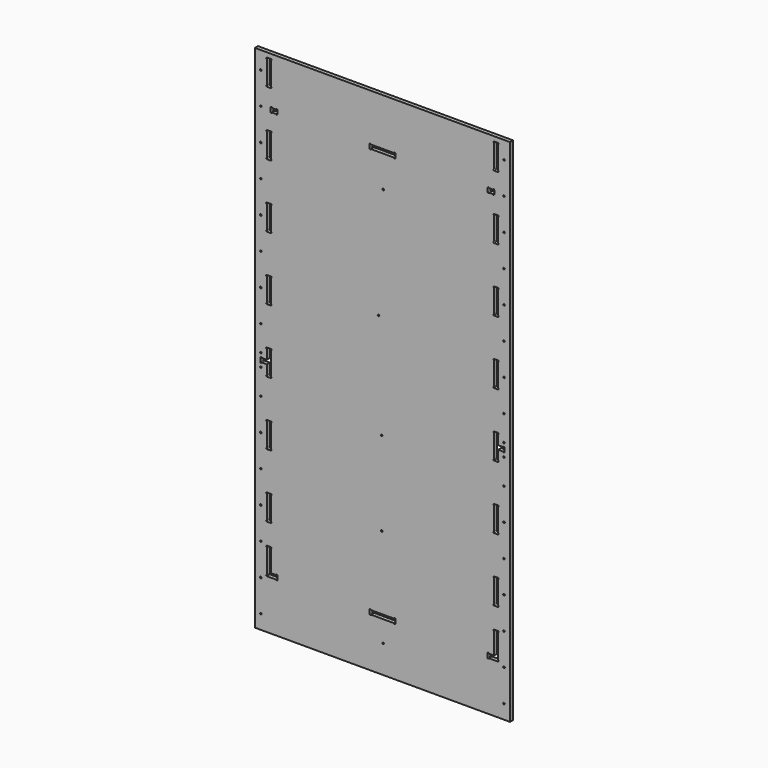
from build123d import *

# Parameters (mm, degrees)
F1_DEPTH = 18


# Not quite as in the source:
# - ends of sketch curves that miss each other by under 0.0002 mm in the source are joined


with BuildPart() as f1:
    # F0 (on Front) → F1 (new body)
    with BuildSketch(Plane.XZ):
        Polygon((-600, 1199.516802), (-600, -1200), (599.475083, -1200), (599.501014, 1199.503749), align=None)
        with BuildLine():
            ThreePointArc((-572.054616, -1136.852261), (-574.7062664294, -1135.7539114294), (-575.804616, -1133.102261))
            ThreePointArc((-575.804616, -1133.102261), (-574.7062664294, -1130.4506105706), (-572.054616, -1129.352261))
            ThreePointArc((-572.054616, -1129.352261), (-569.4029655706, -1130.4506105706), (-568.304616, -1133.102261))
            ThreePointArc((-568.304616, -1133.102261), (-569.4029655706, -1135.7539114294), (-572.054616, -1136.852261))
        make_face(mode=Mode.SUBTRACT)
        with BuildLine():
            ThreePointArc((-572.054616, -986.852261), (-574.7062664294, -985.7539114294), (-575.804616, -983.102261))
            ThreePointArc((-575.804616, -983.102261), (-574.7062664294, -980.4506105706), (-572.054616, -979.352261))
            ThreePointArc((-572.054616, -979.352261), (-569.4029655706, -980.4506105706), (-568.304616, -983.102261))
            ThreePointArc((-568.304616, -983.102261), (-569.4029655706, -985.7539114294), (-572.054616, -986.852261))
        make_face(mode=Mode.SUBTRACT)
        with BuildLine():
            ThreePointArc((-543.7722930308, -848.4810704015), (-546.7808601253, -845.1050301398), (-543.522222, -841.9696830491))
            Line((-543.522222, -841.9696830491), (-525.022204, -841.969884))
            ThreePointArc((-525.022204, -841.969884), (-521.7646201932, -845.1053392321), (-524.7722740702, -848.4812760883))
            Line((-524.7722740702, -848.4812760883), (-524.773356, -949.737518))
            Line((-524.773356, -949.737518), (-500.284715, -949.737785))
            ThreePointArc((-500.284715, -949.737785), (-496.9086751398, -946.7292178747), (-493.7733280491, -949.987856))
            Line((-493.7733280491, -949.987856), (-493.773529, -968.487871))
            ThreePointArc((-493.773529, -968.487871), (-496.9089846919, -971.7454548244), (-500.284921159, -968.7378000122))
            Line((-500.284921159, -968.7378000122), (-543.523601, -968.73733))
            ThreePointArc((-543.523601, -968.73733), (-546.7811848068, -965.6018747679), (-543.7735309298, -962.2259379117))
            Line((-543.7735309298, -962.2259379117), (-543.7722930308, -848.4810704015))
        make_face(mode=Mode.SUBTRACT)
        with BuildLine():
            ThreePointArc((-572.054616, -836.852261), (-574.7062664294, -835.7539114294), (-575.804616, -833.102261))
            ThreePointArc((-575.804616, -833.102261), (-574.7062664294, -830.4506105706), (-572.054616, -829.352261))
            ThreePointArc((-572.054616, -829.352261), (-569.4029655706, -830.4506105706), (-568.304616, -833.102261))
            ThreePointArc((-568.304616, -833.102261), (-569.4029655706, -835.7539114294), (-572.054616, -836.852261))
        make_face(mode=Mode.SUBTRACT)
        with BuildLine():
            ThreePointArc((-572.054616, -686.852261), (-574.7062664294, -685.7539114294), (-575.804616, -683.102261))
            ThreePointArc((-575.804616, -683.102261), (-574.7062664294, -680.4506105706), (-572.054616, -679.352261))
            ThreePointArc((-572.054616, -679.352261), (-569.4029655706, -680.4506105706), (-568.304616, -683.102261))
            ThreePointArc((-568.304616, -683.102261), (-569.4029655706, -685.7539114294), (-572.054616, -686.852261))
        make_face(mode=Mode.SUBTRACT)
        with BuildLine():
            ThreePointArc((-525.019977, -621.9649860431), (-521.7623931741, -625.1004417303), (-524.7700480643, -628.4763781649))
            Line((-524.7700480643, -628.4763781649), (-524.771223, -736.453766))
            ThreePointArc((-524.771223, -736.453766), (-521.7626558747, -739.8298058602), (-525.021294, -742.9651529509))
            Line((-525.021294, -742.9651529509), (-543.521145, -742.964956))
            ThreePointArc((-543.521145, -742.964956), (-546.7787288244, -739.8295003081), (-543.7710740122, -736.453563841))
            Line((-543.7710740122, -736.453563841), (-543.769899, -628.476172))
            ThreePointArc((-543.769899, -628.476172), (-546.7784661253, -625.1001321398), (-543.519828, -621.9647850491))
            Line((-543.519828, -621.9647850491), (-525.019977, -621.9649860431))
        make_face(mode=Mode.SUBTRACT)
        with BuildLine():
            ThreePointArc((-60.7727499569, -949.992565), (-57.6372943081, -946.7349811756), (-54.261357841, -949.7426359878))
            Line((-54.261357841, -949.7426359878), (53.715983, -949.743811))
            ThreePointArc((53.715983, -949.743811), (57.0920228602, -946.7352438747), (60.2273699509, -949.993882))
            Line((60.2273699509, -949.993882), (60.227168, -968.4939))
            ThreePointArc((60.227168, -968.4939), (57.0917123081, -971.7514838244), (53.715775841, -968.7438290122))
            Line((53.715775841, -968.7438290122), (-54.261565, -968.742654))
            ThreePointArc((-54.261565, -968.742654), (-57.6376048602, -971.7512211253), (-60.7729519509, -968.492583))
            Line((-60.7729519509, -968.492583), (-60.7727499569, -949.992565))
        make_face(mode=Mode.SUBTRACT)
        with BuildLine():
            ThreePointArc((-8.115127, -606.325), (-7.0167774294, -603.6733495706), (-4.365127, -602.575))
            ThreePointArc((-4.365127, -602.575), (-1.7134765706, -603.6733495706), (-0.615127, -606.325))
            ThreePointArc((-0.615127, -606.325), (-1.7134765706, -608.9766504294), (-4.365127, -610.075))
            ThreePointArc((-4.365127, -610.075), (-7.0167774294, -608.9766504294), (-8.115127, -606.325))
        make_face(mode=Mode.SUBTRACT)
        with BuildLine():
            ThreePointArc((-572.054616, -536.852261), (-574.7062664294, -535.7539114294), (-575.804616, -533.102261))
            ThreePointArc((-575.804616, -533.102261), (-574.7062664294, -530.4506105706), (-572.054616, -529.352261))
            ThreePointArc((-572.054616, -529.352261), (-569.4029655706, -530.4506105706), (-568.304616, -533.102261))
            ThreePointArc((-568.304616, -533.102261), (-569.4029655706, -535.7539114294), (-572.054616, -536.852261))
        make_face(mode=Mode.SUBTRACT)
        with BuildLine():
            ThreePointArc((-572.054616, -386.852261), (-574.7062664294, -385.7539114294), (-575.804616, -383.102261))
            ThreePointArc((-575.804616, -383.102261), (-574.7062664294, -380.4506105706), (-572.054616, -379.352261))
            ThreePointArc((-572.054616, -379.352261), (-569.4029655706, -380.4506105706), (-568.304616, -383.102261))
            ThreePointArc((-568.304616, -383.102261), (-569.4029655706, -385.7539114294), (-572.054616, -386.852261))
        make_face(mode=Mode.SUBTRACT)
        with BuildLine():
            ThreePointArc((-525.016712, -321.9646860431), (-521.7591281741, -325.1001417303), (-524.7667830643, -328.4760781649))
            Line((-524.7667830643, -328.4760781649), (-524.767958, -436.453466))
            ThreePointArc((-524.767958, -436.453466), (-521.7593908747, -439.8295058602), (-525.018029, -442.9648529509))
            Line((-525.018029, -442.9648529509), (-543.51788, -442.964656))
            ThreePointArc((-543.51788, -442.964656), (-546.7754638244, -439.8292003081), (-543.7678090122, -436.453263841))
            Line((-543.7678090122, -436.453263841), (-543.766634, -328.475872))
            ThreePointArc((-543.766634, -328.475872), (-546.7752011253, -325.0998321398), (-543.516563, -321.9644850491))
            Line((-543.516563, -321.9644850491), (-525.016712, -321.9646860431))
        make_face(mode=Mode.SUBTRACT)
        with BuildLine():
            ThreePointArc((-572.054616, -236.852261), (-574.7062664294, -235.7539114294), (-575.804616, -233.102261))
            ThreePointArc((-575.804616, -233.102261), (-574.7062664294, -230.4506105706), (-572.054616, -229.352261))
            ThreePointArc((-572.054616, -229.352261), (-569.4029655706, -230.4506105706), (-568.304616, -233.102261))
            ThreePointArc((-568.304616, -233.102261), (-569.4029655706, -235.7539114294), (-572.054616, -236.852261))
        make_face(mode=Mode.SUBTRACT)
        with BuildLine():
            ThreePointArc((-572.054616, -116.852261), (-574.7062664294, -115.7539114294), (-575.804616, -113.102261))
            ThreePointArc((-575.804616, -113.102261), (-574.7062664294, -110.4506105706), (-572.054616, -109.352261))
            ThreePointArc((-572.054616, -109.352261), (-569.4029655706, -110.4506105706), (-568.304616, -113.102261))
            ThreePointArc((-568.304616, -113.102261), (-569.4029655706, -115.7539114294), (-572.054616, -116.852261))
        make_face(mode=Mode.SUBTRACT)
        with BuildLine():
            ThreePointArc((-543.514634, -142.9690389274), (-546.7720658527, -139.8334261548), (-543.7642489368, -136.4576348202))
            Line((-543.7642489368, -136.4576348202), (-543.76158, -91.971957))
            Line((-543.76158, -91.971957), (-568.250197, -91.971691))
            ThreePointArc((-568.250197, -91.971691), (-571.6262368602, -94.9802581253), (-574.7615839509, -91.72162))
            Line((-574.7615839509, -91.72162), (-574.761383, -73.221602))
            ThreePointArc((-574.761383, -73.221602), (-571.6259272697, -69.9640181741), (-568.2499908351, -72.9716730643))
            Line((-568.2499908351, -72.9716730643), (-543.761373, -72.971939))
            Line((-543.761373, -72.971939), (-543.763074, -28.480267))
            ThreePointArc((-543.763074, -28.480267), (-546.7718041555, -25.1043722531), (-543.513317, -21.9688680257))
            Line((-543.513317, -21.9688680257), (-525.013448, -21.969069))
            ThreePointArc((-525.013448, -21.969069), (-521.7558641756, -25.1045246919), (-524.7635189878, -28.480461159))
            Line((-524.7635189878, -28.480461159), (-524.764694, -136.457849))
            ThreePointArc((-524.764694, -136.457849), (-521.7561268747, -139.8338888602), (-525.014765, -142.9692359509))
            Line((-525.014765, -142.9692359509), (-543.514634, -142.9690389274))
        make_face(mode=Mode.SUBTRACT)
        with BuildLine():
            ThreePointArc((-572.054616, -56.852261), (-574.7062664294, -55.7539114294), (-575.804616, -53.102261))
            ThreePointArc((-575.804616, -53.102261), (-574.7062664294, -50.4506105706), (-572.054616, -49.352261))
            ThreePointArc((-572.054616, -49.352261), (-569.4029655706, -50.4506105706), (-568.304616, -53.102261))
            ThreePointArc((-568.304616, -53.102261), (-569.4029655706, -55.7539114294), (-572.054616, -56.852261))
        make_face(mode=Mode.SUBTRACT)
        with BuildLine():
            ThreePointArc((-8.115127, -210.239), (-7.0167774294, -207.5873495706), (-4.365127, -206.489))
            ThreePointArc((-4.365127, -206.489), (-1.7134765706, -207.5873495706), (-0.615127, -210.239))
            ThreePointArc((-0.615127, -210.239), (-1.7134765706, -212.8906504294), (-4.365127, -213.989))
            ThreePointArc((-4.365127, -213.989), (-7.0167774294, -212.8906504294), (-8.115127, -210.239))
        make_face(mode=Mode.SUBTRACT)
        with BuildLine():
            ThreePointArc((-0.780127, -1068.426), (0.3182225706, -1065.7743495706), (2.969873, -1064.676))
            ThreePointArc((2.969873, -1064.676), (5.6215234294, -1065.7743495706), (6.719873, -1068.426))
            ThreePointArc((6.719873, -1068.426), (5.6215234294, -1071.0776504294), (2.969873, -1072.176))
            ThreePointArc((2.969873, -1072.176), (0.3182225706, -1071.0776504294), (-0.780127, -1068.426))
        make_face(mode=Mode.SUBTRACT)
        with BuildLine():
            ThreePointArc((571.095767, -1136.852261), (568.4441165706, -1135.7539114294), (567.345767, -1133.102261))
            ThreePointArc((567.345767, -1133.102261), (568.4441165706, -1130.4506105706), (571.095767, -1129.352261))
            ThreePointArc((571.095767, -1129.352261), (573.7474174294, -1130.4506105706), (574.845767, -1133.102261))
            ThreePointArc((574.845767, -1133.102261), (573.7474174294, -1135.7539114294), (571.095767, -1136.852261))
        make_face(mode=Mode.SUBTRACT)
        with BuildLine():
            ThreePointArc((524.2286739692, -848.4939214015), (521.2201068747, -845.1178811398), (524.478745, -841.9825340491))
            Line((524.478745, -841.9825340491), (542.979136, -841.982735))
            ThreePointArc((542.979136, -841.982735), (546.2367198259, -845.1181907303), (543.2290649357, -848.4941271649))
            Line((543.2290649357, -848.4941271649), (543.227828, -962.237769))
            ThreePointArc((543.227828, -962.237769), (546.2363951253, -965.6138088602), (542.977757, -968.7491559509))
            Line((542.977757, -968.7491559509), (499.738725, -968.748685))
            ThreePointArc((499.738725, -968.748685), (496.3626841781, -971.7572521267), (493.2273370491, -968.498614))
            Line((493.2273370491, -968.498614), (493.227539, -949.998596))
            ThreePointArc((493.227539, -949.998596), (496.3629946919, -946.7410121756), (499.738931159, -949.7486669878))
            Line((499.738931159, -949.7486669878), (524.227573, -949.748934))
            Line((524.227573, -949.748934), (524.2286739692, -848.4939214015))
        make_face(mode=Mode.SUBTRACT)
        with BuildLine():
            ThreePointArc((571.095767, -986.852261), (568.4441165706, -985.7539114294), (567.345767, -983.102261))
            ThreePointArc((567.345767, -983.102261), (568.4441165706, -980.4506105706), (571.095767, -979.352261))
            ThreePointArc((571.095767, -979.352261), (573.7474174294, -980.4506105706), (574.845767, -983.102261))
            ThreePointArc((574.845767, -983.102261), (573.7474174294, -985.7539114294), (571.095767, -986.852261))
        make_face(mode=Mode.SUBTRACT)
        with BuildLine():
            ThreePointArc((571.095767, -836.852261), (568.4441165706, -835.7539114294), (567.345767, -833.102261))
            ThreePointArc((567.345767, -833.102261), (568.4441165706, -830.4506105706), (571.095767, -829.352261))
            ThreePointArc((571.095767, -829.352261), (573.7474174294, -830.4506105706), (574.845767, -833.102261))
            ThreePointArc((574.845767, -833.102261), (573.7474174294, -835.7539114294), (571.095767, -836.852261))
        make_face(mode=Mode.SUBTRACT)
        with BuildLine():
            Line((524.230052, -736.46863), (524.231227, -628.49129))
            ThreePointArc((524.231227, -628.49129), (521.2226598747, -625.1152501398), (524.481298, -621.9799030491))
            Line((524.481298, -621.9799030491), (542.981316, -621.980104))
            ThreePointArc((542.981316, -621.980104), (546.2388998259, -625.1155597303), (543.2312449357, -628.4914961649))
            Line((543.2312449357, -628.4914961649), (543.23007, -736.468837))
            ThreePointArc((543.23007, -736.468837), (546.2386371253, -739.8448768602), (542.979999, -742.9802239509))
            Line((542.979999, -742.9802239509), (524.479981, -742.980023))
            ThreePointArc((524.479981, -742.980023), (521.2223971741, -739.8445672697), (524.230052, -736.46863))
        make_face(mode=Mode.SUBTRACT)
        with BuildLine():
            ThreePointArc((571.095767, -686.852261), (568.4441165706, -685.7539114294), (567.345767, -683.102261))
            ThreePointArc((567.345767, -683.102261), (568.4441165706, -680.4506105706), (571.095767, -679.352261))
            ThreePointArc((571.095767, -679.352261), (573.7474174294, -680.4506105706), (574.845767, -683.102261))
            ThreePointArc((574.845767, -683.102261), (573.7474174294, -685.7539114294), (571.095767, -686.852261))
        make_face(mode=Mode.SUBTRACT)
        with BuildLine():
            ThreePointArc((571.095767, -536.852261), (568.4441165706, -535.7539114294), (567.345767, -533.102261))
            ThreePointArc((567.345767, -533.102261), (568.4441165706, -530.4506105706), (571.095767, -529.352261))
            ThreePointArc((571.095767, -529.352261), (573.7474174294, -530.4506105706), (574.845767, -533.102261))
            ThreePointArc((574.845767, -533.102261), (573.7474174294, -535.7539114294), (571.095767, -536.852261))
        make_face(mode=Mode.SUBTRACT)
        with BuildLine():
            ThreePointArc((524.483246, -442.9797229569), (521.2256621741, -439.8442672697), (524.2333170643, -436.4683308351))
            Line((524.2333170643, -436.4683308351), (524.234492, -328.49099))
            ThreePointArc((524.234492, -328.49099), (521.2259238556, -325.114950638), (524.484562, -321.9796030491))
            Line((524.484562, -321.9796030491), (542.98458, -321.979804))
            ThreePointArc((542.98458, -321.979804), (546.2421638068, -325.1152592321), (543.2345099298, -328.4911960883))
            Line((543.2345099298, -328.4911960883), (543.233335, -436.468537))
            ThreePointArc((543.233335, -436.468537), (546.2419021253, -439.8445768602), (542.983264, -442.9799239509))
            Line((542.983264, -442.9799239509), (524.483246, -442.9797229569))
        make_face(mode=Mode.SUBTRACT)
        with BuildLine():
            ThreePointArc((571.095767, -386.852261), (568.4441165706, -385.7539114294), (567.345767, -383.102261))
            ThreePointArc((567.345767, -383.102261), (568.4441165706, -380.4506105706), (571.095767, -379.352261))
            ThreePointArc((571.095767, -379.352261), (573.7474174294, -380.4506105706), (574.845767, -383.102261))
            ThreePointArc((574.845767, -383.102261), (573.7474174294, -385.7539114294), (571.095767, -386.852261))
        make_face(mode=Mode.SUBTRACT)
        with BuildLine():
            ThreePointArc((571.095767, -236.852261), (568.4441165706, -235.7539114294), (567.345767, -233.102261))
            ThreePointArc((567.345767, -233.102261), (568.4441165706, -230.4506105706), (571.095767, -229.352261))
            ThreePointArc((571.095767, -229.352261), (573.7474174294, -230.4506105706), (574.845767, -233.102261))
            ThreePointArc((574.845767, -233.102261), (573.7474174294, -235.7539114294), (571.095767, -236.852261))
        make_face(mode=Mode.SUBTRACT)
        with BuildLine():
            ThreePointArc((524.2377559692, -28.4906904015), (521.2291888747, -25.1146501398), (524.487827, -21.9793030491))
            Line((524.487827, -21.9793030491), (542.987819, -21.979504))
            ThreePointArc((542.987819, -21.979504), (546.2456103474, -25.1147390342), (543.238188986, -28.4908788184))
            Line((543.238188986, -28.4908788184), (543.240772, -72.983768))
            Line((543.240772, -72.983768), (567.729447, -72.984035))
            ThreePointArc((567.729447, -72.984035), (571.105486362, -69.9754668556), (574.2408339509, -73.234105))
            Line((574.2408339509, -73.234105), (574.240633, -91.734123))
            ThreePointArc((574.240633, -91.734123), (571.1051778062, -94.9917068053), (567.7292409176, -91.9840530063))
            Line((567.7292409176, -91.9840530063), (543.240565, -91.983786))
            Line((543.240565, -91.983786), (543.237014, -136.468254))
            ThreePointArc((543.237014, -136.468254), (546.2453486433, -139.8444975193), (542.986502, -142.979623906))
            Line((542.986502, -142.979623906), (524.48651, -142.979423))
            ThreePointArc((524.48651, -142.979423), (521.2289261741, -139.8439672697), (524.2365810643, -136.4680308351))
            Line((524.2365810643, -136.4680308351), (524.2377559692, -28.4906904015))
        make_face(mode=Mode.SUBTRACT)
        with BuildLine():
            ThreePointArc((571.095767, -116.852261), (568.4441165706, -115.7539114294), (567.345767, -113.102261))
            ThreePointArc((567.345767, -113.102261), (568.4441165706, -110.4506105706), (571.095767, -109.352261))
            ThreePointArc((571.095767, -109.352261), (573.7474174294, -110.4506105706), (574.845767, -113.102261))
            ThreePointArc((574.845767, -113.102261), (573.7474174294, -115.7539114294), (571.095767, -116.852261))
        make_face(mode=Mode.SUBTRACT)
        with BuildLine():
            ThreePointArc((571.095767, -56.852261), (568.4441165706, -55.7539114294), (567.345767, -53.102261))
            ThreePointArc((567.345767, -53.102261), (568.4441165706, -50.4506105706), (571.095767, -49.352261))
            ThreePointArc((571.095767, -49.352261), (573.7474174294, -50.4506105706), (574.845767, -53.102261))
            ThreePointArc((574.845767, -53.102261), (573.7474174294, -55.7539114294), (571.095767, -56.852261))
        make_face(mode=Mode.SUBTRACT)
        with BuildLine():
            ThreePointArc((-572.054616, 63.147739), (-574.7062664294, 64.2460885706), (-575.804616, 66.897739))
            ThreePointArc((-575.804616, 66.897739), (-574.7062664294, 69.5493894294), (-572.054616, 70.647739))
            ThreePointArc((-572.054616, 70.647739), (-569.4029655706, 69.5493894294), (-568.304616, 66.897739))
            ThreePointArc((-568.304616, 66.897739), (-569.4029655706, 64.2460885706), (-572.054616, 63.147739))
        make_face(mode=Mode.SUBTRACT)
        with BuildLine():
            ThreePointArc((-572.054616, 213.147739), (-574.7062664294, 214.2460885706), (-575.804616, 216.897739))
            ThreePointArc((-575.804616, 216.897739), (-574.7062664294, 219.5493894294), (-572.054616, 220.647739))
            ThreePointArc((-572.054616, 220.647739), (-569.4029655706, 219.5493894294), (-568.304616, 216.897739))
            ThreePointArc((-568.304616, 216.897739), (-569.4029655706, 214.2460885706), (-572.054616, 213.147739))
        make_face(mode=Mode.SUBTRACT)
        with BuildLine():
            ThreePointArc((-524.7614289692, 163.5471344015), (-521.7528618747, 160.1710941398), (-525.0115, 157.0357470491))
            Line((-525.0115, 157.0357470491), (-543.511351, 157.035943))
            ThreePointArc((-543.511351, 157.035943), (-546.7689348259, 160.1713987303), (-543.7612799357, 163.5473351649))
            Line((-543.7612799357, 163.5473351649), (-543.760105, 271.524728))
            ThreePointArc((-543.760105, 271.524728), (-546.7686721253, 274.9007678602), (-543.510034, 278.0361149509))
            Line((-543.510034, 278.0361149509), (-525.010183, 278.035914))
            ThreePointArc((-525.010183, 278.035914), (-521.7525991741, 274.9004582697), (-524.7602540643, 271.5245218351))
            Line((-524.7602540643, 271.5245218351), (-524.7614289692, 163.5471344015))
        make_face(mode=Mode.SUBTRACT)
        with BuildLine():
            ThreePointArc((-572.054616, 363.147739), (-574.7062664294, 364.2460885706), (-575.804616, 366.897739))
            ThreePointArc((-575.804616, 366.897739), (-574.7062664294, 369.5493894294), (-572.054616, 370.647739))
            ThreePointArc((-572.054616, 370.647739), (-569.4029655706, 369.5493894294), (-568.304616, 366.897739))
            ThreePointArc((-568.304616, 366.897739), (-569.4029655706, 364.2460885706), (-572.054616, 363.147739))
        make_face(mode=Mode.SUBTRACT)
        with BuildLine():
            ThreePointArc((-572.054616, 513.147739), (-574.7062664294, 514.2460885706), (-575.804616, 516.897739))
            ThreePointArc((-575.804616, 516.897739), (-574.7062664294, 519.5493894294), (-572.054616, 520.647739))
            ThreePointArc((-572.054616, 520.647739), (-569.4029655706, 519.5493894294), (-568.304616, 516.897739))
            ThreePointArc((-568.304616, 516.897739), (-569.4029655706, 514.2460885706), (-572.054616, 513.147739))
        make_face(mode=Mode.SUBTRACT)
        with BuildLine():
            ThreePointArc((-525.006919, 578.0362139569), (-521.7493351932, 574.9007587679), (-524.7569890702, 571.5248219117))
            Line((-524.7569890702, 571.5248219117), (-524.758164, 463.547434))
            ThreePointArc((-524.758164, 463.547434), (-521.7495968747, 460.1713941398), (-525.008235, 457.0360470491))
            Line((-525.008235, 457.0360470491), (-543.508086, 457.036243))
            ThreePointArc((-543.508086, 457.036243), (-546.7656698259, 460.1716987303), (-543.7580149357, 463.5476351649))
            Line((-543.7580149357, 463.5476351649), (-543.75684, 571.525028))
            ThreePointArc((-543.75684, 571.525028), (-546.7654081444, 574.901067362), (-543.50677, 578.0364149509))
            Line((-543.50677, 578.0364149509), (-525.006919, 578.0362139569))
        make_face(mode=Mode.SUBTRACT)
        with BuildLine():
            ThreePointArc((-22.784127, 281.201), (-21.6857774294, 283.8526504294), (-19.034127, 284.951))
            ThreePointArc((-19.034127, 284.951), (-16.3824765706, 283.8526504294), (-15.284127, 281.201))
            ThreePointArc((-15.284127, 281.201), (-16.3824765706, 278.5493495706), (-19.034127, 277.451))
            ThreePointArc((-19.034127, 277.451), (-21.6857774294, 278.5493495706), (-22.784127, 281.201))
        make_face(mode=Mode.SUBTRACT)
        with BuildLine():
            ThreePointArc((-572.054616, 663.147739), (-574.7062664294, 664.2460885706), (-575.804616, 666.897739))
            ThreePointArc((-575.804616, 666.897739), (-574.7062664294, 669.5493894294), (-572.054616, 670.647739))
            ThreePointArc((-572.054616, 670.647739), (-569.4029655706, 669.5493894294), (-568.304616, 666.897739))
            ThreePointArc((-568.304616, 666.897739), (-569.4029655706, 664.2460885706), (-572.054616, 663.147739))
        make_face(mode=Mode.SUBTRACT)
        with BuildLine():
            ThreePointArc((-572.054616, 813.147739), (-574.7062664294, 814.2460885706), (-575.804616, 816.897739))
            ThreePointArc((-575.804616, 816.897739), (-574.7062664294, 819.5493894294), (-572.054616, 820.647739))
            ThreePointArc((-572.054616, 820.647739), (-569.4029655706, 819.5493894294), (-568.304616, 816.897739))
            ThreePointArc((-568.304616, 816.897739), (-569.4029655706, 814.2460885706), (-572.054616, 813.147739))
        make_face(mode=Mode.SUBTRACT)
        with BuildLine():
            ThreePointArc((-543.7533610308, 871.5253315985), (-546.7619281253, 874.9013718602), (-543.50329, 878.0367189509))
            Line((-543.50329, 878.0367189509), (-525.003272, 878.036518))
            ThreePointArc((-525.003272, 878.036518), (-521.7456881741, 874.9010622697), (-524.7533430643, 871.5251258351))
            Line((-524.7533430643, 871.5251258351), (-524.754518, 763.547734))
            ThreePointArc((-524.754518, 763.547734), (-521.7459508747, 760.1716941398), (-525.004589, 757.0363470491))
            Line((-525.004589, 757.0363470491), (-543.504607, 757.036548))
            ThreePointArc((-543.504607, 757.036548), (-546.7621908244, 760.1720036919), (-543.7545360122, 763.547940159))
            Line((-543.7545360122, 763.547940159), (-543.7533610308, 871.5253315985))
        make_face(mode=Mode.SUBTRACT)
        with BuildLine():
            ThreePointArc((-572.054616, 963.147739), (-574.7062664294, 964.2460885706), (-575.804616, 966.897739))
            ThreePointArc((-575.804616, 966.897739), (-574.7062664294, 969.5493894294), (-572.054616, 970.647739))
            ThreePointArc((-572.054616, 970.647739), (-569.4029655706, 969.5493894294), (-568.304616, 966.897739))
            ThreePointArc((-568.304616, 966.897739), (-569.4029655706, 964.2460885706), (-572.054616, 963.147739))
        make_face(mode=Mode.SUBTRACT)
        with BuildLine():
            ThreePointArc((-501.2644784015, 977.0329490308), (-497.8884391391, 980.0415161637), (-494.7530910488, 976.78288))
            Line((-494.7530910488, 976.78288), (-494.752949, 958.277954))
            ThreePointArc((-494.752949, 958.277954), (-497.888403196, 955.0203682323), (-501.2643420088, 958.0280219993))
            Line((-501.2643420088, 958.0280219993), (-519.241595, 958.028218))
            ThreePointArc((-519.241595, 958.028218), (-522.6176343606, 955.0196508555), (-525.752981951, 958.278288))
            Line((-525.752981951, 958.278288), (-525.752923, 976.783214))
            ThreePointArc((-525.752923, 976.783214), (-522.6174677679, 980.0407978068), (-519.2415309117, 977.0331439298))
            Line((-519.2415309117, 977.0331439298), (-501.2644784015, 977.0329490308))
        make_face(mode=Mode.SUBTRACT)
        with BuildLine():
            ThreePointArc((-572.054616, 1113.147739), (-574.7062664294, 1114.2460885706), (-575.804616, 1116.897739))
            ThreePointArc((-575.804616, 1116.897739), (-574.7062664294, 1119.5493894294), (-572.054616, 1120.647739))
            ThreePointArc((-572.054616, 1120.647739), (-569.4029655706, 1119.5493894294), (-568.304616, 1116.897739))
            ThreePointArc((-568.304616, 1116.897739), (-569.4029655706, 1114.2460885706), (-572.054616, 1113.147739))
        make_face(mode=Mode.SUBTRACT)
        with BuildLine():
            ThreePointArc((-524.7515879633, 1063.5478364778), (-521.7430198556, 1060.171796638), (-525.001658, 1057.0364490491))
            Line((-525.001658, 1057.0364490491), (-543.501509, 1057.036651))
            ThreePointArc((-543.501509, 1057.036651), (-546.7590928244, 1060.1721066919), (-543.7514380122, 1063.548043159))
            Line((-543.7514380122, 1063.548043159), (-543.750263, 1171.525431))
            ThreePointArc((-543.750263, 1171.525431), (-546.7588311444, 1174.901470362), (-543.500193, 1178.0368179509))
            Line((-543.500193, 1178.0368179509), (-525.000342, 1178.036621))
            ThreePointArc((-525.000342, 1178.036621), (-521.7427581932, 1174.9011657679), (-524.7504120702, 1171.5252289117))
            Line((-524.7504120702, 1171.5252289117), (-524.7515879633, 1063.5478364778))
        make_face(mode=Mode.SUBTRACT)
        with BuildLine():
            ThreePointArc((53.7365535985, 977.0268890308), (57.1125928609, 980.0354561637), (60.2479409512, 976.77682))
            Line((60.2479409512, 976.77682), (60.248139, 958.276642))
            ThreePointArc((60.248139, 958.276642), (57.1126843059, 955.0190572139), (53.7367469176, 958.0267109937))
            Line((53.7367469176, 958.0267109937), (-54.240597, 958.027886))
            ThreePointArc((-54.240597, 958.027886), (-57.6166358624, 955.0193178364), (-60.751983951, 958.277955))
            Line((-60.751983951, 958.277955), (-60.751982, 976.778133))
            ThreePointArc((-60.751982, 976.778133), (-57.6165273059, 980.0357177861), (-54.2405899176, 977.0280640063))
            Line((-54.2405899176, 977.0280640063), (53.7365535985, 977.0268890308))
        make_face(mode=Mode.SUBTRACT)
        with BuildLine():
            ThreePointArc((571.095767, 63.147739), (568.4441165706, 64.2460885706), (567.345767, 66.897739))
            ThreePointArc((567.345767, 66.897739), (568.4441165706, 69.5493894294), (571.095767, 70.647739))
            ThreePointArc((571.095767, 70.647739), (573.7474174294, 69.5493894294), (574.845767, 66.897739))
            ThreePointArc((574.845767, 66.897739), (573.7474174294, 64.2460885706), (571.095767, 63.147739))
        make_face(mode=Mode.SUBTRACT)
        with BuildLine():
            ThreePointArc((524.489775, 157.0208770431), (521.2321911741, 160.1563327303), (524.2398460643, 163.5322691649))
            Line((524.2398460643, 163.5322691649), (524.241021, 271.50961))
            ThreePointArc((524.241021, 271.50961), (521.2324538747, 274.8856498602), (524.491092, 278.0209969509))
            Line((524.491092, 278.0209969509), (542.99111, 278.020796))
            ThreePointArc((542.99111, 278.020796), (546.2486938259, 274.8853402697), (543.2410389357, 271.5094038351))
            Line((543.2410389357, 271.5094038351), (543.239864, 163.532063))
            ThreePointArc((543.239864, 163.532063), (546.2484311253, 160.1560231398), (542.989793, 157.0206760491))
            Line((542.989793, 157.0206760491), (524.489775, 157.0208770431))
        make_face(mode=Mode.SUBTRACT)
        with BuildLine():
            ThreePointArc((571.095767, 213.147739), (568.4441165706, 214.2460885706), (567.345767, 216.897739))
            ThreePointArc((567.345767, 216.897739), (568.4441165706, 219.5493894294), (571.095767, 220.647739))
            ThreePointArc((571.095767, 220.647739), (573.7474174294, 219.5493894294), (574.845767, 216.897739))
            ThreePointArc((574.845767, 216.897739), (573.7474174294, 214.2460885706), (571.095767, 213.147739))
        make_face(mode=Mode.SUBTRACT)
        with BuildLine():
            ThreePointArc((571.095767, 363.147739), (568.4441165706, 364.2460885706), (567.345767, 366.897739))
            ThreePointArc((567.345767, 366.897739), (568.4441165706, 369.5493894294), (571.095767, 370.647739))
            ThreePointArc((571.095767, 370.647739), (573.7474174294, 369.5493894294), (574.845767, 366.897739))
            ThreePointArc((574.845767, 366.897739), (573.7474174294, 364.2460885706), (571.095767, 363.147739))
        make_face(mode=Mode.SUBTRACT)
        with BuildLine():
            ThreePointArc((524.493039, 457.0211770431), (521.2354551741, 460.1566327303), (524.2431100643, 463.5325691649))
            Line((524.2431100643, 463.5325691649), (524.244285, 571.50991))
            ThreePointArc((524.244285, 571.50991), (521.2357178747, 574.8859498602), (524.494356, 578.0212969509))
            Line((524.494356, 578.0212969509), (542.994374, 578.021096))
            ThreePointArc((542.994374, 578.021096), (546.2519578259, 574.8856402697), (543.2443029357, 571.5097038351))
            Line((543.2443029357, 571.5097038351), (543.243128, 463.532363))
            ThreePointArc((543.243128, 463.532363), (546.2516951253, 460.1563231398), (542.993057, 457.0209760491))
            Line((542.993057, 457.0209760491), (524.493039, 457.0211770431))
        make_face(mode=Mode.SUBTRACT)
        with BuildLine():
            ThreePointArc((571.095767, 513.147739), (568.4441165706, 514.2460885706), (567.345767, 516.897739))
            ThreePointArc((567.345767, 516.897739), (568.4441165706, 519.5493894294), (571.095767, 520.647739))
            ThreePointArc((571.095767, 520.647739), (573.7474174294, 519.5493894294), (574.845767, 516.897739))
            ThreePointArc((574.845767, 516.897739), (573.7474174294, 514.2460885706), (571.095767, 513.147739))
        make_face(mode=Mode.SUBTRACT)
        with BuildLine():
            ThreePointArc((-0.780127, 809.315), (0.3182225706, 811.9666504294), (2.969873, 813.065))
            ThreePointArc((2.969873, 813.065), (5.6215234294, 811.9666504294), (6.719873, 809.315))
            ThreePointArc((6.719873, 809.315), (5.6215234294, 806.6633495706), (2.969873, 805.565))
            ThreePointArc((2.969873, 805.565), (0.3182225706, 806.6633495706), (-0.780127, 809.315))
        make_face(mode=Mode.SUBTRACT)
        with BuildLine():
            ThreePointArc((571.095767, 663.147739), (568.4441165706, 664.2460885706), (567.345767, 666.897739))
            ThreePointArc((567.345767, 666.897739), (568.4441165706, 669.5493894294), (571.095767, 670.647739))
            ThreePointArc((571.095767, 670.647739), (573.7474174294, 669.5493894294), (574.845767, 666.897739))
            ThreePointArc((574.845767, 666.897739), (573.7474174294, 664.2460885706), (571.095767, 663.147739))
        make_face(mode=Mode.SUBTRACT)
        with BuildLine():
            ThreePointArc((524.496304, 757.0214770431), (521.2387201741, 760.1569327303), (524.2463750643, 763.5328691649))
            Line((524.2463750643, 763.5328691649), (524.24755, 871.51021))
            ThreePointArc((524.24755, 871.51021), (521.2389828747, 874.8862498602), (524.497621, 878.0215969509))
            Line((524.497621, 878.0215969509), (542.997639, 878.021396))
            ThreePointArc((542.997639, 878.021396), (546.2552228259, 874.8859402697), (543.2475679357, 871.5100038351))
            Line((543.2475679357, 871.5100038351), (543.246393, 763.532663))
            ThreePointArc((543.246393, 763.532663), (546.2549601253, 760.1566231398), (542.996322, 757.0212760491))
            Line((542.996322, 757.0212760491), (524.496304, 757.0214770431))
        make_face(mode=Mode.SUBTRACT)
        with BuildLine():
            ThreePointArc((571.095767, 813.147739), (568.4441165706, 814.2460885706), (567.345767, 816.897739))
            ThreePointArc((567.345767, 816.897739), (568.4441165706, 819.5493894294), (571.095767, 820.647739))
            ThreePointArc((571.095767, 820.647739), (573.7474174294, 819.5493894294), (574.845767, 816.897739))
            ThreePointArc((574.845767, 816.897739), (573.7474174294, 814.2460885706), (571.095767, 813.147739))
        make_face(mode=Mode.SUBTRACT)
        with BuildLine():
            ThreePointArc((525.2483379569, 958.271581), (522.1128827679, 955.0139971932), (518.7369459117, 958.0216510702))
            Line((518.7369459117, 958.0216510702), (500.759692, 958.021846))
            ThreePointArc((500.759692, 958.021846), (497.3836521398, 955.0132788747), (494.2483050491, 958.271917))
            Line((494.2483050491, 958.271917), (494.248523, 976.772078))
            ThreePointArc((494.248523, 976.772078), (497.3839786919, 980.0296618244), (500.759915159, 977.0220070122))
            Line((500.759915159, 977.0220070122), (518.736978, 977.021812))
            ThreePointArc((518.736978, 977.021812), (522.1130173606, 980.0303791445), (525.248364951, 976.771742))
            Line((525.248364951, 976.771742), (525.2483379569, 958.271581))
        make_face(mode=Mode.SUBTRACT)
        with BuildLine():
            ThreePointArc((571.095767, 963.147739), (568.4441165706, 964.2460885706), (567.345767, 966.897739))
            ThreePointArc((567.345767, 966.897739), (568.4441165706, 969.5493894294), (571.095767, 970.647739))
            ThreePointArc((571.095767, 970.647739), (573.7474174294, 969.5493894294), (574.845767, 966.897739))
            ThreePointArc((574.845767, 966.897739), (573.7474174294, 964.2460885706), (571.095767, 963.147739))
        make_face(mode=Mode.SUBTRACT)
        with BuildLine():
            ThreePointArc((543.2494770308, 1063.5329634015), (546.2580441253, 1060.1569231398), (542.999406, 1057.0215760491))
            Line((542.999406, 1057.0215760491), (524.499584, 1057.021777))
            ThreePointArc((524.499584, 1057.021777), (521.2420001756, 1060.1572326919), (524.2496549878, 1063.533169159))
            Line((524.2496549878, 1063.533169159), (524.25083, 1171.51051))
            ThreePointArc((524.25083, 1171.51051), (521.2422628747, 1174.8865498602), (524.500901, 1178.0218969509))
            Line((524.500901, 1178.0218969509), (543.000723, 1178.021696))
            ThreePointArc((543.000723, 1178.021696), (546.2583068259, 1174.8862402697), (543.2506519357, 1171.5103038351))
            Line((543.2506519357, 1171.5103038351), (543.2494770308, 1063.5329634015))
        make_face(mode=Mode.SUBTRACT)
        with BuildLine():
            ThreePointArc((571.095767, 1113.147739), (568.4441165706, 1114.2460885706), (567.345767, 1116.897739))
            ThreePointArc((567.345767, 1116.897739), (568.4441165706, 1119.5493894294), (571.095767, 1120.647739))
            ThreePointArc((571.095767, 1120.647739), (573.7474174294, 1119.5493894294), (574.845767, 1116.897739))
            ThreePointArc((574.845767, 1116.897739), (573.7474174294, 1114.2460885706), (571.095767, 1113.147739))
        make_face(mode=Mode.SUBTRACT)
    extrude(amount=F1_DEPTH)


solid = f1.part
